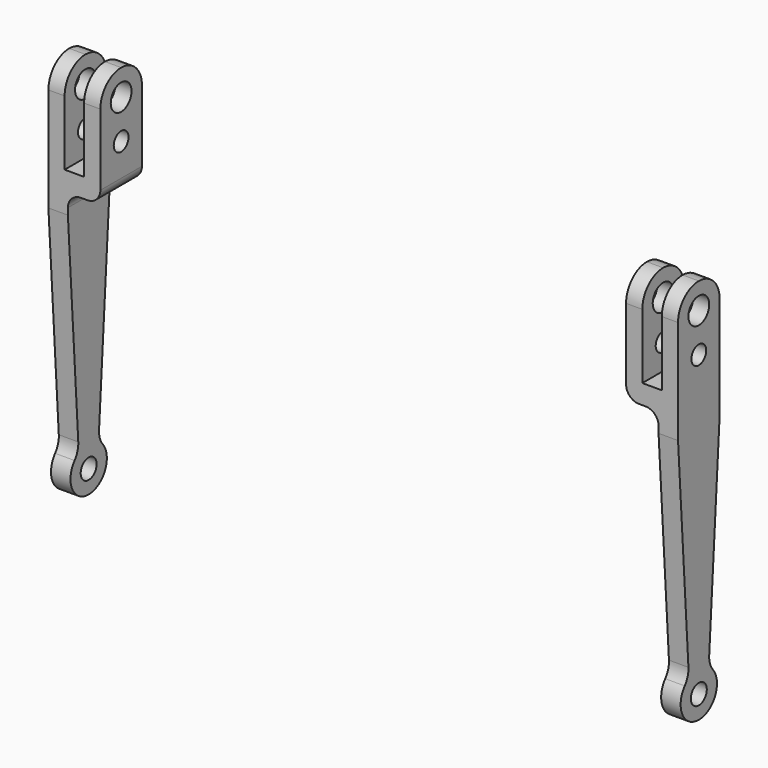
from build123d import *

# Parameters (mm, degrees)
F1_DEPTH = 6.35
F2_R     = 1.5875
F3_R     = 3.17499
F5_D     = 3.175
F7_D     = 2.2606
F8_R     = 1.2192
F9_DEPTH = 25.4


# Not quite as in the source:
# - a fillet or chamfer is up to 0.001 mm smaller than in the source, because OpenCascade refuses the exact size


with BuildPart() as f1:
    # F0 (on Front) → F1 (new body)
    with BuildSketch(Plane.XZ):
        Polygon((36.1012686809, 4.7600296621), (38.4825186809, 4.7600296621), (38.4825186809, 51.9881546621), (36.4981436809, 51.9881546621), (36.4981436809, 40.8756546621), (34.1168936809, 40.8756546621), (34.1168936809, 51.9881546621), (32.1325186809, 51.9881546621), (32.1325186809, 38.4944046621), (36.1012686809, 38.4944046621), align=None)
    extrude(amount=F1_DEPTH)

    # F2
    f2_edges = [f1.edges().sort_by_distance(p)[0] for p in [
        (36.101269, -3.175, 38.494405),
        (32.132519, -3.175, 38.494405),
    ]]
    fillet(f2_edges, radius=F2_R)

    # F3 (radius 3.175 in the source; OpenCascade refuses exactly that, so slightly less here)
    f3_edges = [f1.edges().sort_by_distance(p)[0] for p in [
        (33.124706, -6.35, 51.988155),
        (33.124706, 0, 51.988155),
        (37.490331, 0, 51.988155),
        (37.490331, -6.35, 51.988155),
    ]]
    fillet(f3_edges, radius=F3_R)

    # F5 (through all)
    with Locations(Plane.YZ.offset(38.4825186809)):
        with Locations((-3.175, 48.8131546621)):
            Hole(F5_D / 2)

    # F7 (through all)
    with Locations(Plane.YZ.offset(38.4825186809)):
        with Locations((-3.175, 44.0506546621)):
            Hole(F7_D / 2)

    # F8 (on face) → F9 (cut)
    with BuildSketch(Plane.YZ.offset(38.4825186809)):
        Polygon((-6.35, 11.0568078235), (-4.7625, 11.0568078235), (-6.35, 36.1131546621), align=None)
        with BuildLine():
            Line((-6.35, 4.7600296621), (-3.175, 4.7600296621))
            ThreePointArc((-3.175, 4.7600296621), (-5.684534213, 6.3464262746), (-5.3280227481, 9.2938515499))
            ThreePointArc((-5.3280227481, 9.2938515499), (-4.8786206586, 10.1218745235), (-4.7625, 11.0568078235))
            Line((-4.7625, 11.0568078235), (-6.35, 11.0568078235))
            Line((-6.35, 11.0568078235), (-6.35, 4.7600296621))
        make_face()
        with Locations((-3.175, 7.5381546621)):
            Circle(F8_R)
        with BuildLine():
            ThreePointArc((-1.0219772519, 9.2938515499), (-0.5578121163, 8.4699840975), (-0.396875, 7.5381546621))
            ThreePointArc((-0.396875, 7.5381546621), (-1.2105689735, 5.5737236356), (-3.175, 4.7600296621))
            Line((-3.175, 4.7600296621), (0, 4.7600296621))
            Line((0, 4.7600296621), (0, 11.0568078235))
            Line((0, 11.0568078235), (-1.5875, 11.0568078235))
            ThreePointArc((-1.5875, 11.0568078235), (-1.4713793414, 10.1218745235), (-1.0219772519, 9.2938515499))
        make_face()
        Polygon((0, 36.1131546621), (-1.5875, 11.0568078235), (0, 11.0568078235), align=None)
    extrude(amount=-F9_DEPTH, mode=Mode.SUBTRACT)


with BuildPart() as f11_1:
    # F11: instance of F1
    add(f1.part.mirror(Plane.YZ))


solid = Compound([f1.part, f11_1.part])
